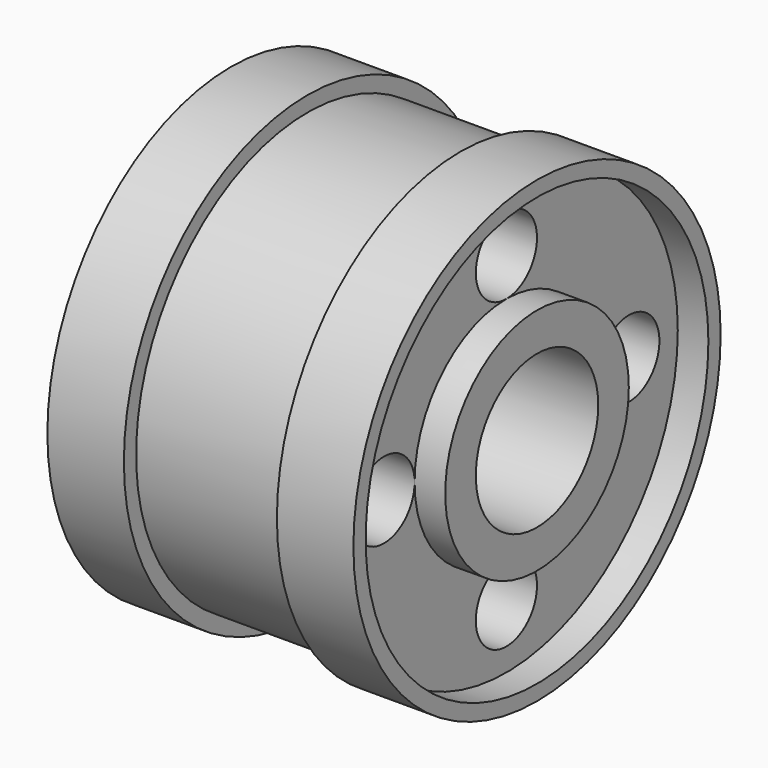
from build123d import *

# Parameters (mm, degrees)
F2_R     = 2.5
F3_DEPTH = 20.001
F5_R     = 14
F5_R_2   = 7.5
F6_DEPTH = 3
F8_R     = 14
F8_R_2   = 7.5
F9_DEPTH = 3


with BuildPart() as f1:
    # F0 (on Top) → F1 (revolve)
    with BuildSketch(Plane.XY):
        Polygon((12.0361039788, 5), (12.0361039788, 15), (7.0361039788, 15), (7.0361039788, 14), (-2.9638960212, 14), (-2.9638960212, 15), (-7.9638960212, 15), (-7.9638960212, 5), align=None)
    revolve(axis=Axis((-2.1188026294, 0, 0), (1, 0, 0)))

    # F2 (on face) → F3 (cut, through all)
    with BuildSketch(Plane(origin=(-7.9638960212, 0, 0), x_dir=(0, -1, 0), z_dir=(-1, 0, 0))):
        with Locations((-10, 0)):
            Circle(F2_R)
        with Locations((10, 0)):
            Circle(F2_R)
        with Locations((0, 10)):
            Circle(F2_R)
        with Locations((0, -10)):
            Circle(F2_R)
    extrude(amount=-F3_DEPTH, mode=Mode.SUBTRACT)

    # F5 (on offset) → F6 (cut)
    with BuildSketch(Plane(origin=(-8.9638960212, 0, 0), x_dir=(0, -1, 0), z_dir=(-1, 0, 0))):
        Circle(F5_R)
        Circle(F5_R_2, mode=Mode.SUBTRACT)
    extrude(amount=-F6_DEPTH, mode=Mode.SUBTRACT)

    # F8 (on offset) → F9 (cut)
    with BuildSketch(Plane.YZ.offset(13.0361039788)):
        Circle(F8_R)
        Circle(F8_R_2, mode=Mode.SUBTRACT)
    extrude(amount=-F9_DEPTH, mode=Mode.SUBTRACT)


solid = f1.part
